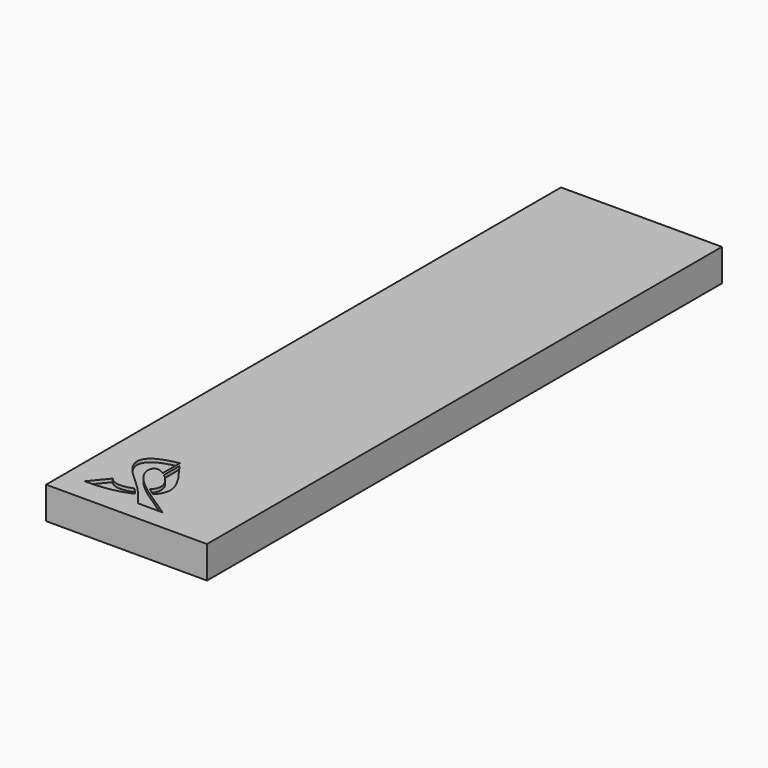
from build123d import *

# Parameters (mm, degrees)
F0_W     = 200
F0_H     = 800
F1_DEPTH = 40
F3_DEPTH = 4


# Not quite as in the source:
# - ends of sketch curves that miss each other by under 0.0002 mm in the source are joined
# - a feature of the source that left no trace in its solid (it failed there, or was rolled back) is left out


with BuildPart() as f1:
    # F0 (on Top) → F1 (new body)
    with BuildSketch(Plane.XY):
        with Locations((100, 400)):
            Rectangle(F0_W, F0_H)
    extrude(amount=-F1_DEPTH)

    # F2 (on face) → F3 (cut)
    with BuildSketch(Plane.XY):
        with BuildLine():
            add(Edge.make_bspline(
                [(74.0144076195, 49.4648806587), (79.2780666431, 43.995087588), (85.5330334882, 36.6035044423), (93.9858326346, 24.9514187131)],
                knots=[0, 0, 0, 0, 1, 1, 1, 1], degree=3))
            Line((93.9858326346, 24.9514187131), (124.8743034899, 24.9514187131))
            add(Edge.make_bspline(
                [(124.8743034899, 24.9514187131), (117.373795502, 30.8557542171), (100.1070204646, 40.4994924549), (85.0477587545, 51.6157174292)],
                knots=[0, 0, 0, 0, 1, 1, 1, 1], degree=3))
            add(Edge.make_bspline(
                [(85.0477587545, 51.6157174292), (78.3221982923, 56.5802620007), (72.0369383461, 61.8389475301), (67.2585806524, 67.1891107778)],
                knots=[0, 0, 0, 0, 1, 1, 1, 1], degree=3))
            add(Edge.make_bspline(
                [(67.2585806524, 67.1891107778), (64.0111017086, 70.825439839), (61.4596060965, 74.5036446576), (59.9390200859, 78.1614235749)],
                knots=[0, 0, 0, 0, 1, 1, 1, 1], degree=3))
            add(Edge.make_bspline(
                [(59.9390200859, 78.1614235749), (58.6848351698, 81.1781536647), (58.1318996379, 84.1804553021), (58.4680892286, 87.1331416805)],
                knots=[0, 0, 0, 0, 1, 1, 1, 1], degree=3))
            add(Edge.make_bspline(
                [(58.4680892286, 87.1331416805), (58.8494259124, 90.279355495), (60.7095393399, 92.4826134262), (63.6064002406, 92.9386057154)],
                knots=[0, 0, 0, 0, 1, 1, 1, 1], degree=3))
            add(Edge.make_bspline(
                [(63.6064002406, 92.9386057154), (66.1469914002, 93.338307093), (69.4850038962, 92.3950054588), (73.3222940387, 89.5654596054)],
                knots=[0, 0, 0, 0, 1, 1, 1, 1], degree=3))
            Line((73.3222940387, 89.5654596054), (73.3850611313, 116.1375625051))
            add(Edge.make_bspline(
                [(73.3850611313, 116.1375625051), (61.2635786151, 114.5669223978), (16.5941537425, 105.3232312885), (51.4149430547, 70.5446634846)],
                knots=[0, 0, 0, 0, 1, 1, 1, 1], degree=3))
            add(Edge.make_bspline(
                [(51.4149430547, 70.5446634846), (59.7059440621, 62.0496960224), (65.5907579364, 58.2180974722), (74.0144076195, 49.4648806587)],
                knots=[0, 0, 0, 0, 1, 1, 1, 1], degree=3))
        make_face()
        with BuildLine():
            add(Edge.make_bspline(
                [(91.6621868878, 90.8201365516), (86.9476734338, 98.0875153234), (81.3030633718, 105.4382865607), (76.6022868683, 111.646603626)],
                knots=[0, 0, 0, 0, 1, 1, 1, 1], degree=3))
            Line((76.6022868683, 111.646603626), (76.7011849335, 87.2598062052))
            add(Edge.make_bspline(
                [(76.7011849335, 87.2598062052), (83.8706497004, 81.3502046486), (97.2544954721, 67.4086626207), (84.6318469774, 55.4167037236)],
                knots=[0, 0, 0, 0, 1, 1, 1, 1], degree=3))
            add(Edge.make_bspline(
                [(84.6318469774, 55.4167037236), (87.753206619, 52.954491641), (90.1454573299, 51.1927975466), (93.6734466659, 48.8385927365)],
                knots=[0, 0, 0, 0, 1, 1, 1, 1], degree=3))
            add(Edge.make_bspline(
                [(93.6734466659, 48.8385927365), (99.7215214715, 54.7664924964), (102.6407232018, 62.4339183966), (101.2052451133, 70.0858652935)],
                knots=[0, 0, 0, 0, 1, 1, 1, 1], degree=3))
            add(Edge.make_bspline(
                [(101.2052451133, 70.0858652935), (100.3360804582, 76.0348691585), (96.4859975312, 83.3838717469), (91.6621868878, 90.8201365516)],
                knots=[0, 0, 0, 0, 1, 1, 1, 1], degree=3))
        make_face()
        with BuildLine():
            add(Edge.make_bspline(
                [(71.9907407021, 47.2640828783), (51.4723643059, 39.233897758), (44.7548226057, 48.169378506), (42.5680809306, 50.3631415847)],
                knots=[0, 0, 0, 0, 1, 1, 1, 1], degree=3))
            Line((42.5680809306, 50.3631415847), (24.8743034899, 28.961757198))
            add(Edge.make_bspline(
                [(24.8743034899, 28.961757198), (35.1755403208, 28.6025219778), (57.6930087218, 28.8069538664), (79.2330525311, 38.8320952786)],
                knots=[0, 0, 0, 0, 1, 1, 1, 1], degree=3))
            add(Edge.make_bspline(
                [(79.2330525311, 38.8320952786), (77.1638794716, 41.6785297354), (74.3423390821, 44.7962323959), (71.9907407021, 47.2640828783)],
                knots=[0, 0, 0, 0, 1, 1, 1, 1], degree=3))
        make_face()
    extrude(amount=-F3_DEPTH, mode=Mode.SUBTRACT)


solid = f1.part
